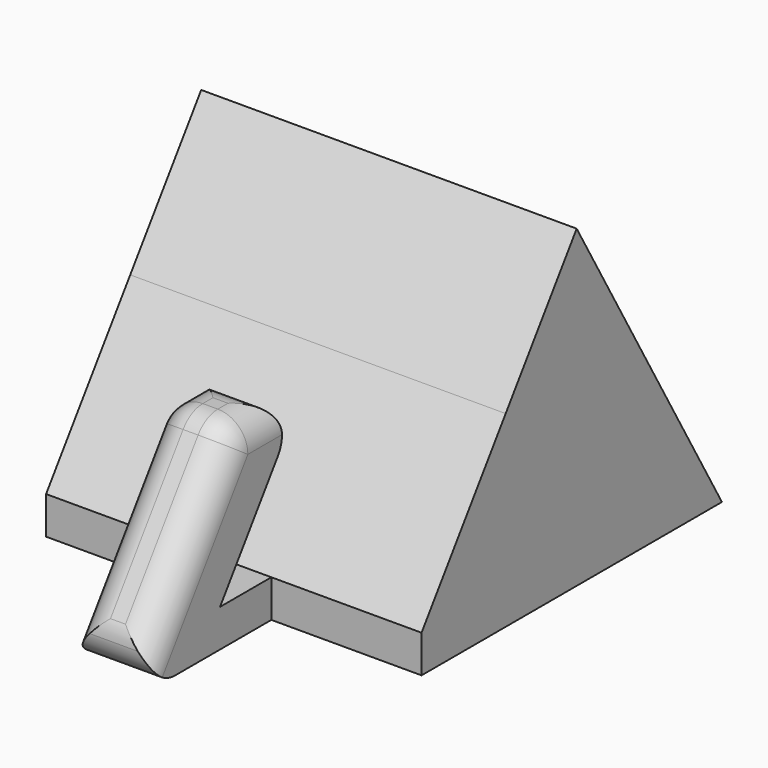
from build123d import *

# Parameters (mm, degrees)
F1_DEPTH      = 5
F2_DEPTH      = 25
F2_DEPTH_BACK = 25
F3_T1_DEPTH   = 32.333223573
F3_T3_DEPTH   = 16.3059757776
F3_T5_DEPTH   = 2
F3_T7_DEPTH   = 48.4196425394
F3_T9_DEPTH   = 30
F3_T14_DEPTH  = 4.08
F3_T20_DEPTH  = 4.08
F3_T26_DEPTH  = 19.3723096765
F3_T31_DEPTH  = 19.3723096765


# Not quite as in the source:
# - a fillet or chamfer that OpenCascade refuses, or shapes differently, is made with other operations: its cross-section is extruded or revolved along the edge and cut away or added


with BuildPart() as f1:
    # F0 (on Right) → F1 (new body, symmetric)
    with BuildSketch(Plane.YZ):
        Polygon((0, 0), (0, 5), (-8.5454221213, 5), (5.4587286429, 25), (-5.9958492358, 25), (-20, 5), (-20, 0), align=None)
    extrude(amount=F1_DEPTH, both=True)

    # F0 (on Right) → F2 (join, two sides)
    with BuildSketch(Plane.YZ) as f2_sk:
        Polygon((14.0041507642, 25), (0, 5), (0, 0), (50, 0), (25.8219641147, 41.8775865806), align=None)
    extrude(amount=F2_DEPTH)
    extrude(f2_sk.sketch, amount=-F2_DEPTH_BACK)

    # F3: fillet of radius 4 on 8 edges, made by hand

    # F3_s2 → F3_t1 (cut)
    with BuildSketch(Plane(origin=(0, 8.5792437745, 12.2524298959), x_dir=(1, 0, 0), z_dir=(0, -0.5735764364, -0.8191520443))):
        with BuildLine():
            ThreePointArc((-5, 15.2509230675), (-3.8284271247, 18.0793501923), (-1, 19.2509230675))
            Line((-1, 19.2509230675), (-5, 19.2509230675))
            Line((-5, 19.2509230675), (-5, 15.2509230675))
        make_face()
        with BuildLine():
            ThreePointArc((5, 15.2509230675), (3.8284271247, 18.0793501923), (1, 19.2509230675))
            Line((1, 19.2509230675), (5, 19.2509230675))
            Line((5, 19.2509230675), (5, 15.2509230675))
        make_face()
    extrude(amount=F3_T1_DEPTH, mode=Mode.SUBTRACT)

    # F3_s4 → F3_t3 (cut)
    with BuildSketch(Plane.YZ.offset(-8.1529878888)):
        with BuildLine():
            ThreePointArc((-19.2766081772, 6.0331105899), (-19.814867803, 4.9416280425), (-20, 3.7388048445))
            Line((-20, 3.7388048445), (-20, 5))
            Line((-20, 5), (-19.2766081772, 6.0331105899))
        make_face()
    extrude(amount=F3_T3_DEPTH, mode=Mode.SUBTRACT)

    # F3_s6 → F3_t5 (cut)
    with BuildSketch(Plane.YZ.offset(-1)):
        with BuildLine():
            ThreePointArc((-7.1901892108, 23.2943057454), (-5.7605754865, 24.5480433327), (-3.9135810336, 25))
            Line((-3.9135810336, 25), (-5.9958492358, 25))
            Line((-5.9958492358, 25), (-7.1901892108, 23.2943057454))
        make_face()
    extrude(amount=F3_T5_DEPTH, mode=Mode.SUBTRACT)

    # F3_s8 → F3_t7 (cut)
    with BuildSketch(Plane.YZ.offset(-24.2098212697)):
        with BuildLine():
            ThreePointArc((1.0514083121, 18.7056942546), (1.3228434677, 22.8469944529), (-2.225199865, 25))
            Line((-2.225199865, 25), (5.4587286429, 25))
            Line((5.4587286429, 25), (1.0514083121, 18.7056942546))
        make_face()
    extrude(amount=F3_T7_DEPTH, mode=Mode.SUBTRACT)

    # F3_s10 → F3_t9 (cut)
    with BuildSketch(Plane.YZ.offset(-15)):
        with BuildLine():
            ThreePointArc((-16, 0), (-18.8284271247, 1.1715728753), (-20, 4))
            Line((-20, 4), (-20, 0))
            Line((-20, 0), (-16, 0))
        make_face()
    extrude(amount=F3_T9_DEPTH, mode=Mode.SUBTRACT)


with BuildPart() as f3_tool12:
    # F3_s13 → F3_t14 (new body)
    with BuildSketch(Plane.YZ.offset(-1)):
        Polygon((-3.9135810336, 21), (-7.2557213743, 23.3401918603), (-6.0374945998, 25.08), (-3.9135810336, 25.08), align=None)
    extrude(amount=-F3_T14_DEPTH)

    # F3_s15 → F3_t16 (revolve, cut)
    with BuildSketch(Plane(origin=(-1, -3.9135810336, 21), x_dir=(0, 0.4617486132, -0.8870108332), z_dir=(0, 0.8870108332, 0.4617486132))):
        with BuildLine():
            ThreePointArc((0, -4), (4, 0), (0, 4))
            Line((0, 4), (0, -4))
        make_face()
    revolve(axis=Axis((-1, -3.9135810336, 21), (-1, 0, 0)), mode=Mode.SUBTRACT)


with BuildPart() as f1_1:
    add(f1.part)

    # F3_t11: cut F3_tool12
    add(f3_tool12.part, mode=Mode.SUBTRACT)


with BuildPart() as f3_tool18:
    # F3_s19 → F3_t20 (new body)
    with BuildSketch(Plane.YZ.offset(1)):
        Polygon((-3.9135810336, 21), (-7.2557213743, 23.3401918603), (-6.0374945998, 25.08), (-3.9135810336, 25.08), align=None)
    extrude(amount=F3_T20_DEPTH)

    # F3_s21 → F3_t22 (revolve, cut)
    with BuildSketch(Plane(origin=(1, -3.9135810336, 21), x_dir=(0, 0.4617486132, -0.8870108332), z_dir=(0, -0.8870108332, -0.4617486132))):
        with BuildLine():
            ThreePointArc((0, -4), (4, 0), (0, 4))
            Line((0, 4), (0, -4))
        make_face()
    revolve(axis=Axis((1, -3.9135810336, 21), (1, 0, 0)), mode=Mode.SUBTRACT)


with BuildPart() as f1_2:
    add(f1_1.part)

    # F3_t17: cut F3_tool18
    add(f3_tool18.part, mode=Mode.SUBTRACT)


with BuildPart() as f3_tool24:
    # F3_s25 → F3_t26 (new body)
    with BuildSketch(Plane.XZ.offset(-15.4587286429)):
        with BuildLine():
            ThreePointArc((-5, 21), (-3.8284271247, 23.8284271247), (-1, 25))
            Line((-1, 25), (-5, 25))
            Line((-5, 25), (-5, 21))
        make_face()
    extrude(amount=F3_T26_DEPTH)

    split(bisect_by=Plane(origin=(0, -8.083295862, 5.6599846961), x_dir=(1, 0, 0), z_dir=(0, -0.8191520443, 0.5735764364)), keep=Keep.TOP)


with BuildPart() as f1_3:
    add(f1_2.part)

    # F3_t23: cut F3_tool24
    add(f3_tool24.part, mode=Mode.SUBTRACT)


with BuildPart() as f3_tool29:
    # F3_s30 → F3_t31 (new body)
    with BuildSketch(Plane.XZ.offset(-15.4587286429)):
        with BuildLine():
            ThreePointArc((5, 21), (3.8284271247, 23.8284271247), (1, 25))
            Line((1, 25), (5, 25))
            Line((5, 25), (5, 21))
        make_face()
    extrude(amount=F3_T31_DEPTH)

    split(bisect_by=Plane(origin=(0, -8.083295862, 5.6599846961), x_dir=(1, 0, 0), z_dir=(0, -0.8191520443, 0.5735764364)), keep=Keep.TOP)


with BuildPart() as f1_4:
    add(f1_3.part)

    # F3_t28: cut F3_tool29
    add(f3_tool29.part, mode=Mode.SUBTRACT)


solid = f1_4.part
